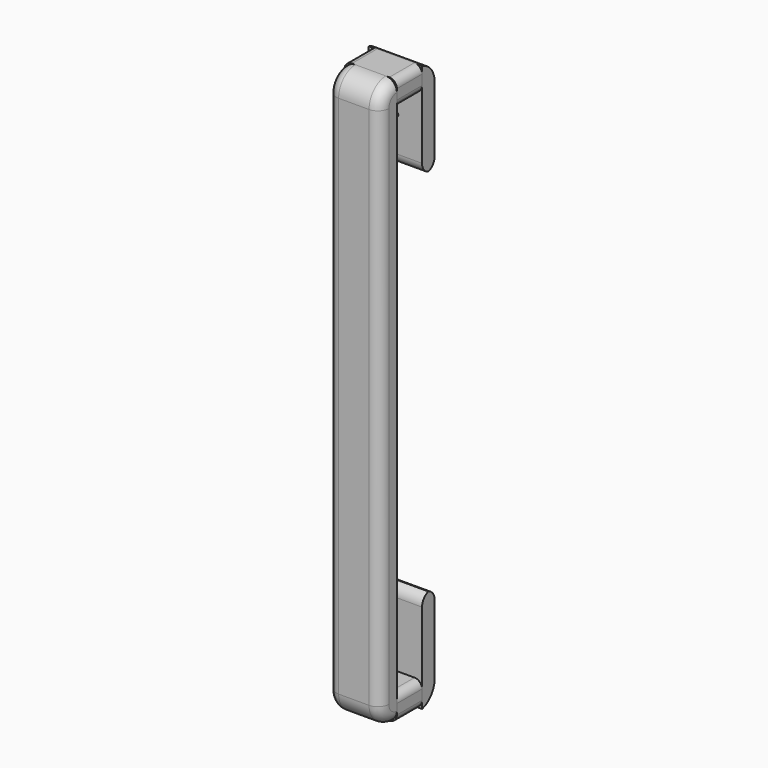
from build123d import *

# Parameters (mm, degrees)
F1_DEPTH      = 7.62
F0_W          = 6.35
F0_H          = 124.968
F2_DEPTH      = 5.08
F3_W          = 12.7
F3_H          = 6.096
F4_DEPTH      = 3.81
F3_W_2        = 12.9487617709
F3_H_2        = 23.389633745
F6_DEPTH      = 25.4
F7_F1_R       = 5.0799
F7_F2_R       = 5.0799
F7_2_T1_DEPTH = 37.5422060193
F7_3_T1_DEPTH = 37.5422060193
F8_F1_R       = 2.6664988796
F8_F2_R       = 2.6664988796
F8_2_T1_DEPTH = 26.2812561691
F8_3_T1_DEPTH = 26.2812561691
F9_R          = 1.8309637078
F9_2_R        = 1.8309637078


# Not quite as in the source:
# - a fillet or chamfer that OpenCascade refuses, or shapes differently, is made with other operations: its cross-section is extruded or revolved along the edge and cut away or added
# - a fillet or chamfer is up to 0.001 mm smaller than in the source, because OpenCascade refuses the exact size


with BuildPart() as f1:
    # F0 (on Front) → F1 (new body)
    with BuildSketch(Plane.XZ):
        Polygon((0, -62.484), (-6.35, -62.484), (-6.35, -68.58), (6.35, -68.58), (6.35, -62.484), align=None)
    extrude(amount=-F1_DEPTH)

    # F9
    f9_edges = [f1.edges().sort_by_distance(p)[0] for p in [
        (6.35, 3.81, -68.58),
        (6.35, 3.81, -62.484),
        (-6.35, 3.81, -62.484),
        (-6.35, 3.81, -68.58),
    ]]
    fillet(f9_edges, radius=F9_R)


with BuildPart() as f1b:
    # F0 (on Front) → F1, piece 2 (new body)
    with BuildSketch(Plane.XZ):
        Polygon((6.35, 68.58), (-6.35, 68.58), (-6.35, 62.484), (0, 62.484), (6.35, 62.484), align=None)
    extrude(amount=-F1_DEPTH)

    # F9#2
    f9_2_edges = [f1b.edges().sort_by_distance(p)[0] for p in [
        (6.35, 3.81, 68.58),
        (-6.35, 3.81, 68.58),
        (6.35, 3.81, 62.484),
        (-6.35, 3.81, 62.484),
    ]]
    fillet(f9_2_edges, radius=F9_2_R)


with BuildPart() as f2:
    # F0 (on Front) → F2 (new body)
    with BuildSketch(Plane.XZ):
        with Locations((3.175, 0)):
            Rectangle(F0_W, F0_H)
        with Locations((-3.175, 0)):
            Rectangle(F0_W, F0_H)
        Polygon((0, -62.484), (-6.35, -62.484), (-6.35, -68.58), (6.35, -68.58), (6.35, -62.484), align=None)
        Polygon((6.35, 68.58), (-6.35, 68.58), (-6.35, 62.484), (0, 62.484), (6.35, 62.484), align=None)
    extrude(amount=F2_DEPTH)

    # F7: fillet of radius 5.08 on 2 edges, made by hand

    # F7_f1 (radius 5.08 in the source; OpenCascade refuses exactly that, so slightly less here)
    f7_f1_edges = [f2.edges().sort_by_distance(p)[0] for p in [
        (0, -5.08, -68.58),
    ]]
    fillet(f7_f1_edges, radius=F7_F1_R)

    # F7_f2 (radius 5.08 in the source; OpenCascade refuses exactly that, so slightly less here)
    f7_f2_edges = [f2.edges().sort_by_distance(p)[0] for p in [
        (0, -5.08, 68.58),
    ]]
    fillet(f7_f2_edges, radius=F7_F2_R)

    # F8: fillet of radius 2.6664988796 on 10 edges, made by hand

    # F8_f1
    f8_f1_edges = [f2.edges().sort_by_distance(p)[0] for p in [
        (-6.35, -5.08, 0),
        (-6.35, -3.5921317377, 67.0921317377),
        (-6.35, -3.5921317377, -67.0921317377),
        (-6.35, -5e-05, 68.58),
        (-6.35, -5e-05, -68.58),
    ]]
    fillet(f8_f1_edges, radius=F8_F1_R)

    # F8_f2
    f8_f2_edges = [f2.edges().sort_by_distance(p)[0] for p in [
        (6.35, -5.08, 0),
        (6.35, -3.5921317377, 67.0921317377),
        (6.35, -3.5921317377, -67.0921317377),
        (6.35, -5e-05, 68.58),
        (6.35, -5e-05, -68.58),
    ]]
    fillet(f8_f2_edges, radius=F8_F2_R)


with BuildPart() as f4:
    # F3 (on face) → F4 (new body)
    with BuildSketch(Plane(origin=(0, 7.62, 0), x_dir=(-1, 0, 0), z_dir=(0, 1, 0))):
        Polygon((6.35, -62.484), (6.35, -68.58), (6.5987617709, -68.58), (6.5987617709, -44.1940687597), (-6.35, -44.1940687597), (-6.35, -62.484), align=None)
        with Locations((0, -65.532)):
            Rectangle(F3_W, F3_H)
    extrude(amount=F4_DEPTH)

    # F7#2: fillet of radius 5.08 on 1 edges, made by hand

    # F7_2_s2 → F7_2_t1 (cut)
    with BuildSketch(Plane.YZ.offset(-18.8954838951)):
        with BuildLine():
            ThreePointArc((7.62, -68.58), (10.3660926284, -66.7721631237), (11.43, -63.6613111503))
            Line((11.43, -63.6613111503), (11.43, -68.58))
            Line((11.43, -68.58), (7.62, -68.58))
        make_face()
    extrude(amount=F7_2_T1_DEPTH, mode=Mode.SUBTRACT)

    # F8#2: fillet of radius 2.6664988796 on 2 edges, made by hand

    # F8_2_s2 → F8_2_t1 (cut)
    with BuildSketch(Plane.YZ.offset(-13.26500897)):
        with BuildLine():
            ThreePointArc((8.7635011204, -44.1940687597), (10.6490005602, -44.9750681995), (11.43, -46.8605676393))
            Line((11.43, -46.8605676393), (11.43, -44.1940687597))
            Line((11.43, -44.1940687597), (8.7635011204, -44.1940687597))
        make_face()
        with BuildLine():
            ThreePointArc((7.62, -46.8605676393), (8.4009994398, -44.9750681995), (10.2864988796, -44.1940687597))
            Line((10.2864988796, -44.1940687597), (7.62, -44.1940687597))
            Line((7.62, -44.1940687597), (7.62, -46.8605676393))
        make_face()
    extrude(amount=F8_2_T1_DEPTH, mode=Mode.SUBTRACT)


with BuildPart() as f4b:
    # F3 (on face) → F4, piece 2 (new body)
    with BuildSketch(Plane(origin=(0, 7.62, 0), x_dir=(-1, 0, 0), z_dir=(0, 1, 0))):
        with Locations((0.1243808854, 56.7673463374)):
            Rectangle(F3_W_2, F3_H_2)
    extrude(amount=F4_DEPTH)

    # F5 (on face) → F6 (cut)
    with BuildSketch(Plane(origin=(0, 11.43, 0), x_dir=(-1, 0, 0), z_dir=(0, 1, 0))):
        with BuildLine():
            ThreePointArc((0.0093760507, 56.7322248993), (-0.427566153, 55.7113620808), (0.6, 56.1322981624))
            ThreePointArc((0.6, 56.1322981624), (0.427566153, 56.553234244), (0.0093760507, 56.7322248993))
        make_face()
    extrude(amount=-F6_DEPTH, mode=Mode.SUBTRACT)

    # F7#3: fillet of radius 5.08 on 1 edges, made by hand

    # F7_3_s2 → F7_3_t1 (cut)
    with BuildSketch(Plane.YZ.offset(-18.8954838951)):
        with BuildLine():
            ThreePointArc((7.62, 68.4621632099), (10.3660926284, 66.6543263336), (11.43, 63.5434743602))
            Line((11.43, 63.5434743602), (11.43, 68.4621632099))
            Line((11.43, 68.4621632099), (7.62, 68.4621632099))
        make_face()
    extrude(amount=F7_3_T1_DEPTH, mode=Mode.SUBTRACT)

    # F8#3: fillet of radius 2.6664988796 on 2 edges, made by hand

    # F8_3_s2 → F8_3_t1 (cut)
    with BuildSketch(Plane.YZ.offset(-13.26500897)):
        with BuildLine():
            ThreePointArc((8.7635011204, 45.072529465), (10.6490005602, 45.8535289048), (11.43, 47.7390283446))
            Line((11.43, 47.7390283446), (11.43, 45.072529465))
            Line((11.43, 45.072529465), (8.7635011204, 45.072529465))
        make_face()
        with BuildLine():
            ThreePointArc((7.62, 47.7390283446), (8.4009994398, 45.8535289048), (10.2864988796, 45.072529465))
            Line((10.2864988796, 45.072529465), (7.62, 45.072529465))
            Line((7.62, 45.072529465), (7.62, 47.7390283446))
        make_face()
    extrude(amount=F8_3_T1_DEPTH, mode=Mode.SUBTRACT)


solid = Compound([f1.part, f1b.part, f2.part, f4.part, f4b.part])
